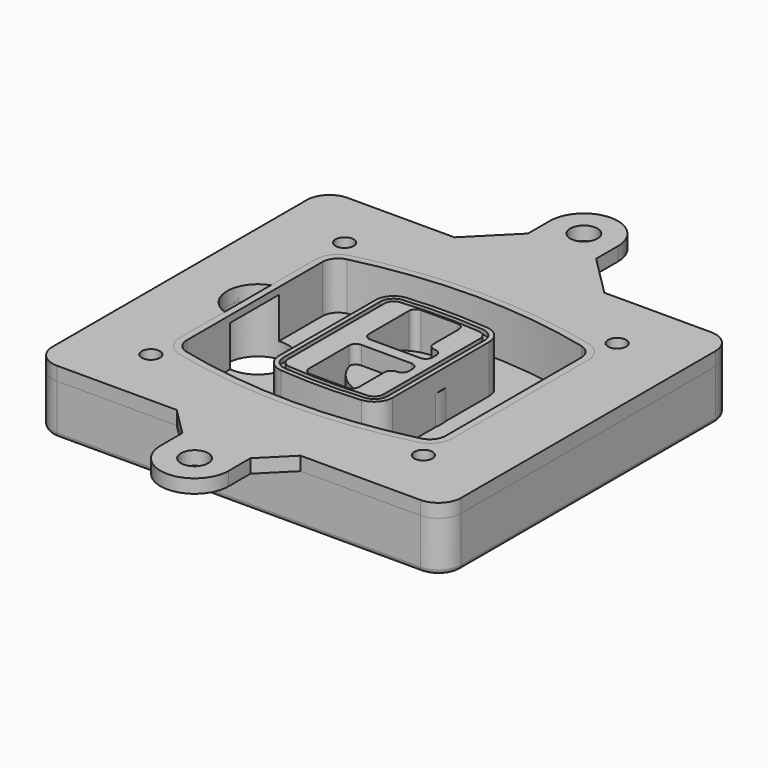
from build123d import *

# Parameters (mm, degrees)
F0_R      = 4
F1_DEPTH  = 25
F2_DEPTH  = 3
F3_DEPTH  = 18
F5_DEPTH  = 21
F6_DEPTH  = 2
F8_DEPTH  = 20
F9_DEPTH  = 16
F10_DEPTH = 25
F7_R      = 6
F7_R_2    = 4
F11_DEPTH = 6
F13_DEPTH = 9
F15_R     = 2
F16_R     = 4
F17_DEPTH = 3


# Not quite as in the source:
# - a feature of the source that left no trace in its solid (it failed there, or was rolled back) is left out
# - a feature names something its author has since deleted; it is built from what else it names


with BuildPart() as f1:
    # F0 (on Top) → F1 (new body)
    with BuildSketch(Plane.XY):
        with BuildLine():
            ThreePointArc((-90, -70), (-87.0710678119, -77.0710678119), (-80, -80))
            Line((-80, -80), (80, -80))
            ThreePointArc((80, -80), (87.0710678119, -77.0710678119), (90, -70))
            Line((90, -70), (90, 70))
            ThreePointArc((90, 70), (87.0710678119, 77.0710678119), (80, 80))
            Line((80, 80), (-80, 80))
            ThreePointArc((-80, 80), (-87.0710678119, 77.0710678119), (-90, 70))
            Line((-90, 70), (-90, -70))
        make_face()
        with Locations((-60, -53.3333333333)):
            Circle(F0_R, mode=Mode.SUBTRACT)
        with Locations((60, -53.3333333333)):
            Circle(F0_R, mode=Mode.SUBTRACT)
        with Locations((-60, 53.3333333333)):
            Circle(F0_R, mode=Mode.SUBTRACT)
        with BuildLine():
            ThreePointArc((-64, 37.2990447398), (-61.0143011354, 45.9411029726), (-53.3306899286, 50.8970778549))
            ThreePointArc((-53.3306899286, 50.8970778549), (0, 57.3333333333), (53.3306899286, 50.8970778549))
            ThreePointArc((53.3306899286, 50.8970778549), (61.0143011354, 45.9411029726), (64, 37.2990447398))
            Line((64, 37.2990447398), (64, -37.2990447398))
            ThreePointArc((64, -37.2990447398), (61.0143011354, -45.9411029726), (53.3306899286, -50.8970778549))
            ThreePointArc((53.3306899286, -50.8970778549), (0, -57.3333333333), (-53.3306899286, -50.8970778549))
            ThreePointArc((-53.3306899286, -50.8970778549), (-61.0143011354, -45.9411029726), (-64, -37.2990447398))
            Line((-64, -37.2990447398), (-64, 37.2990447398))
        make_face(mode=Mode.SUBTRACT)
        with Locations((60, 53.3333333333)):
            Circle(F0_R, mode=Mode.SUBTRACT)
        with BuildLine():
            ThreePointArc((53.3306899286, 50.8970778549), (0, 57.3333333333), (-53.3306899286, 50.8970778549))
            ThreePointArc((-53.3306899286, 50.8970778549), (-61.0143011354, 45.9411029726), (-64, 37.2990447398))
            Line((-64, 37.2990447398), (-64, -37.2990447398))
            ThreePointArc((-64, -37.2990447398), (-61.0143011354, -45.9411029726), (-53.3306899286, -50.8970778549))
            ThreePointArc((-53.3306899286, -50.8970778549), (0, -57.3333333333), (53.3306899286, -50.8970778549))
            ThreePointArc((53.3306899286, -50.8970778549), (61.0143011354, -45.9411029726), (64, -37.2990447398))
            Line((64, -37.2990447398), (64, 37.2990447398))
            ThreePointArc((64, 37.2990447398), (61.0143011354, 45.9411029726), (53.3306899286, 50.8970778549))
        make_face()
        with BuildLine():
            Line((-60, -37.2990447398), (-60, 37.2990447398))
            ThreePointArc((-60, 37.2990447398), (-57.8673579538, 43.4719434775), (-52.3790642347, 47.0119255363))
            ThreePointArc((-52.3790642347, 47.0119255363), (0, 53.3333333333), (52.3790642347, 47.0119255363))
            ThreePointArc((52.3790642347, 47.0119255363), (57.8673579538, 43.4719434775), (60, 37.2990447398))
            Line((60, 37.2990447398), (60, -37.2990447398))
            ThreePointArc((60, -37.2990447398), (57.8673579538, -43.4719434775), (52.3790642347, -47.0119255363))
            ThreePointArc((52.3790642347, -47.0119255363), (0, -53.3333333333), (-52.3790642347, -47.0119255363))
            ThreePointArc((-52.3790642347, -47.0119255363), (-57.8673579538, -43.4719434775), (-60, -37.2990447398))
        make_face(mode=Mode.SUBTRACT)
        with BuildLine():
            ThreePointArc((-52.3790642347, 47.0119255363), (-57.8673579538, 43.4719434775), (-60, 37.2990447398))
            Line((-60, 37.2990447398), (-60, -37.2990447398))
            ThreePointArc((-60, -37.2990447398), (-57.8673579538, -43.4719434775), (-52.3790642347, -47.0119255363))
            ThreePointArc((-52.3790642347, -47.0119255363), (0, -53.3333333333), (52.3790642347, -47.0119255363))
            ThreePointArc((52.3790642347, -47.0119255363), (57.8673579538, -43.4719434775), (60, -37.2990447398))
            Line((60, -37.2990447398), (60, 37.2990447398))
            ThreePointArc((60, 37.2990447398), (57.8673579538, 43.4719434775), (52.3790642347, 47.0119255363))
            ThreePointArc((52.3790642347, 47.0119255363), (0, 53.3333333333), (-52.3790642347, 47.0119255363))
        make_face()
        with BuildLine():
            ThreePointArc((51.6653449643, 44.0980612973), (55.5071505677, 41.6200738562), (57, 37.2990447398))
            Line((57, 37.2990447398), (57, -37.2990447398))
            ThreePointArc((57, -37.2990447398), (55.5071505677, -41.6200738562), (51.6653449643, -44.0980612973))
            ThreePointArc((51.6653449643, -44.0980612973), (0, -50.3333333333), (-51.6653449643, -44.0980612973))
            ThreePointArc((-51.6653449643, -44.0980612973), (-55.5071505677, -41.6200738562), (-57, -37.2990447398))
            Line((-57, -37.2990447398), (-57, 37.2990447398))
            ThreePointArc((-57, 37.2990447398), (-55.5071505677, 41.6200738562), (-51.6653449643, 44.0980612973))
            ThreePointArc((-51.6653449643, 44.0980612973), (0, 50.3333333333), (51.6653449643, 44.0980612973))
        make_face(mode=Mode.SUBTRACT)
        with BuildLine():
            Line((57, -37.2990447398), (57, 37.2990447398))
            ThreePointArc((57, 37.2990447398), (55.5071505677, 41.6200738562), (51.6653449643, 44.0980612973))
            ThreePointArc((51.6653449643, 44.0980612973), (0, 50.3333333333), (-51.6653449643, 44.0980612973))
            ThreePointArc((-51.6653449643, 44.0980612973), (-55.5071505677, 41.6200738562), (-57, 37.2990447398))
            Line((-57, 37.2990447398), (-57, -37.2990447398))
            ThreePointArc((-57, -37.2990447398), (-55.5071505677, -41.6200738562), (-51.6653449643, -44.0980612973))
            ThreePointArc((-51.6653449643, -44.0980612973), (0, -50.3333333333), (51.6653449643, -44.0980612973))
            ThreePointArc((51.6653449643, -44.0980612973), (55.5071505677, -41.6200738562), (57, -37.2990447398))
        make_face()
    extrude(amount=-F1_DEPTH)

    # F0 (on Top) → F2 (join)
    with BuildSketch(Plane.XY):
        with BuildLine():
            ThreePointArc((-52.3790642347, 47.0119255363), (-57.8673579538, 43.4719434775), (-60, 37.2990447398))
            Line((-60, 37.2990447398), (-60, -37.2990447398))
            ThreePointArc((-60, -37.2990447398), (-57.8673579538, -43.4719434775), (-52.3790642347, -47.0119255363))
            ThreePointArc((-52.3790642347, -47.0119255363), (0, -53.3333333333), (52.3790642347, -47.0119255363))
            ThreePointArc((52.3790642347, -47.0119255363), (57.8673579538, -43.4719434775), (60, -37.2990447398))
            Line((60, -37.2990447398), (60, 37.2990447398))
            ThreePointArc((60, 37.2990447398), (57.8673579538, 43.4719434775), (52.3790642347, 47.0119255363))
            ThreePointArc((52.3790642347, 47.0119255363), (0, 53.3333333333), (-52.3790642347, 47.0119255363))
        make_face()
        with BuildLine():
            ThreePointArc((51.6653449643, 44.0980612973), (55.5071505677, 41.6200738562), (57, 37.2990447398))
            Line((57, 37.2990447398), (57, -37.2990447398))
            ThreePointArc((57, -37.2990447398), (55.5071505677, -41.6200738562), (51.6653449643, -44.0980612973))
            ThreePointArc((51.6653449643, -44.0980612973), (0, -50.3333333333), (-51.6653449643, -44.0980612973))
            ThreePointArc((-51.6653449643, -44.0980612973), (-55.5071505677, -41.6200738562), (-57, -37.2990447398))
            Line((-57, -37.2990447398), (-57, 37.2990447398))
            ThreePointArc((-57, 37.2990447398), (-55.5071505677, 41.6200738562), (-51.6653449643, 44.0980612973))
            ThreePointArc((-51.6653449643, 44.0980612973), (0, 50.3333333333), (51.6653449643, 44.0980612973))
        make_face(mode=Mode.SUBTRACT)
    extrude(amount=F2_DEPTH)

    # F0 (on Top) → F3 (cut)
    with BuildSketch(Plane.XY):
        with BuildLine():
            Line((57, -37.2990447398), (57, 37.2990447398))
            ThreePointArc((57, 37.2990447398), (55.5071505677, 41.6200738562), (51.6653449643, 44.0980612973))
            ThreePointArc((51.6653449643, 44.0980612973), (0, 50.3333333333), (-51.6653449643, 44.0980612973))
            ThreePointArc((-51.6653449643, 44.0980612973), (-55.5071505677, 41.6200738562), (-57, 37.2990447398))
            Line((-57, 37.2990447398), (-57, -37.2990447398))
            ThreePointArc((-57, -37.2990447398), (-55.5071505677, -41.6200738562), (-51.6653449643, -44.0980612973))
            ThreePointArc((-51.6653449643, -44.0980612973), (0, -50.3333333333), (51.6653449643, -44.0980612973))
            ThreePointArc((51.6653449643, -44.0980612973), (55.5071505677, -41.6200738562), (57, -37.2990447398))
        make_face()
    extrude(amount=-F3_DEPTH, mode=Mode.SUBTRACT)

    # F4 (on face) → F5 (join, through all)
    with BuildSketch(Plane.XY.offset(3)):
        with BuildLine():
            ThreePointArc((-25, -26.587695628), (-22.8992979869, -31.9912392117), (-17.7004291845, -34.5569740744))
            ThreePointArc((-17.7004291845, -34.5569740744), (0, -35.3333333333), (17.7004291845, -34.5569740744))
            ThreePointArc((17.7004291845, -34.5569740744), (22.8992979869, -31.9912392117), (25, -26.587695628))
            Line((25, -26.587695628), (25, 26.587695628))
            ThreePointArc((25, 26.587695628), (22.8992979869, 31.9912392117), (17.7004291845, 34.5569740744))
            ThreePointArc((17.7004291845, 34.5569740744), (0, 35.3333333333), (-17.7004291845, 34.5569740744))
            ThreePointArc((-17.7004291845, 34.5569740744), (-22.8992979869, 31.9912392117), (-25, 26.587695628))
            Line((-25, 26.587695628), (-25, -26.587695628))
        make_face()
        with BuildLine():
            ThreePointArc((17.5253218884, 32.5646544628), (21.4244734902, 30.6403533158), (23, 26.587695628))
            Line((23, 26.587695628), (23, -26.587695628))
            ThreePointArc((23, -26.587695628), (21.4244734902, -30.6403533158), (17.5253218884, -32.5646544628))
            ThreePointArc((17.5253218884, -32.5646544628), (0, -33.3333333333), (-17.5253218884, -32.5646544628))
            ThreePointArc((-17.5253218884, -32.5646544628), (-21.4244734902, -30.6403533158), (-23, -26.587695628))
            Line((-23, -26.587695628), (-23, 26.587695628))
            ThreePointArc((-23, 26.587695628), (-21.4244734902, 30.6403533158), (-17.5253218884, 32.5646544628))
            ThreePointArc((-17.5253218884, 32.5646544628), (0, 33.3333333333), (17.5253218884, 32.5646544628))
        make_face(mode=Mode.SUBTRACT)
        with BuildLine():
            Line((23, -26.587695628), (23, 26.587695628))
            ThreePointArc((23, 26.587695628), (21.4244734902, 30.6403533158), (17.5253218884, 32.5646544628))
            ThreePointArc((17.5253218884, 32.5646544628), (0, 33.3333333333), (-17.5253218884, 32.5646544628))
            ThreePointArc((-17.5253218884, 32.5646544628), (-21.4244734902, 30.6403533158), (-23, 26.587695628))
            Line((-23, 26.587695628), (-23, -26.587695628))
            ThreePointArc((-23, -26.587695628), (-21.4244734902, -30.6403533158), (-17.5253218884, -32.5646544628))
            ThreePointArc((-17.5253218884, -32.5646544628), (0, -33.3333333333), (17.5253218884, -32.5646544628))
            ThreePointArc((17.5253218884, -32.5646544628), (21.4244734902, -30.6403533158), (23, -26.587695628))
        make_face()
        with BuildLine():
            ThreePointArc((17.3502145923, 30.5723348512), (19.9496489934, 29.2894674198), (21, 26.587695628))
            Line((21, 26.587695628), (21, -26.587695628))
            ThreePointArc((21, -26.587695628), (19.9496489934, -29.2894674198), (17.3502145923, -30.5723348512))
            ThreePointArc((17.3502145923, -30.5723348512), (0, -31.3333333333), (-17.3502145923, -30.5723348512))
            ThreePointArc((-17.3502145923, -30.5723348512), (-19.9496489934, -29.2894674198), (-21, -26.587695628))
            Line((-21, -26.587695628), (-21, 26.587695628))
            ThreePointArc((-21, 26.587695628), (-19.9496489934, 29.2894674198), (-17.3502145923, 30.5723348512))
            ThreePointArc((-17.3502145923, 30.5723348512), (0, 31.3333333333), (17.3502145923, 30.5723348512))
        make_face(mode=Mode.SUBTRACT)
        with BuildLine():
            Line((21, -26.587695628), (21, 26.587695628))
            ThreePointArc((21, 26.587695628), (19.9496489934, 29.2894674198), (17.3502145923, 30.5723348512))
            ThreePointArc((17.3502145923, 30.5723348512), (0, 31.3333333333), (-17.3502145923, 30.5723348512))
            ThreePointArc((-17.3502145923, 30.5723348512), (-19.9496489934, 29.2894674198), (-21, 26.587695628))
            Line((-21, 26.587695628), (-21, -26.587695628))
            ThreePointArc((-21, -26.587695628), (-19.9496489934, -29.2894674198), (-17.3502145923, -30.5723348512))
            ThreePointArc((-17.3502145923, -30.5723348512), (0, -31.3333333333), (17.3502145923, -30.5723348512))
            ThreePointArc((17.3502145923, -30.5723348512), (19.9496489934, -29.2894674198), (21, -26.587695628))
        make_face()
        with BuildLine():
            Line((-8, -2.5), (14, -2.5))
            ThreePointArc((14, -2.5), (16.1213203436, -3.3786796564), (17, -5.5))
            Line((17, -5.5), (17, -7.5))
            ThreePointArc((17, -7.5), (16.1213203436, -9.6213203436), (14, -10.5))
            ThreePointArc((14, -10.5), (11.8786796564, -11.3786796564), (11, -13.5))
            Line((11, -13.5), (11, -27.5))
            ThreePointArc((11, -27.5), (10.1213203436, -29.6213203436), (8, -30.5))
            Line((8, -30.5), (-8, -30.5))
            ThreePointArc((-8, -30.5), (-10.1213203436, -29.6213203436), (-11, -27.5))
            Line((-11, -27.5), (-11, -5.5))
            ThreePointArc((-11, -5.5), (-10.1213203436, -3.3786796564), (-8, -2.5))
        make_face(mode=Mode.SUBTRACT)
        with BuildLine():
            ThreePointArc((-8, 2.5), (-10.1213203436, 3.3786796564), (-11, 5.5))
            Line((-11, 5.5), (-11, 27.5))
            ThreePointArc((-11, 27.5), (-10.1213203436, 29.6213203436), (-8, 30.5))
            Line((-8, 30.5), (8, 30.5))
            ThreePointArc((8, 30.5), (10.1213203436, 29.6213203436), (11, 27.5))
            Line((11, 27.5), (11, 13.5))
            ThreePointArc((11, 13.5), (11.8786796564, 11.3786796564), (14, 10.5))
            ThreePointArc((14, 10.5), (16.1213203436, 9.6213203436), (17, 7.5))
            Line((17, 7.5), (17, 5.5))
            ThreePointArc((17, 5.5), (16.1213203436, 3.3786796564), (14, 2.5))
            Line((14, 2.5), (-8, 2.5))
        make_face(mode=Mode.SUBTRACT)
    extrude(amount=-F5_DEPTH)

    # F4 (on face) → F6 (cut)
    with BuildSketch(Plane.XY.offset(3)):
        with BuildLine():
            Line((23, -26.587695628), (23, 26.587695628))
            ThreePointArc((23, 26.587695628), (21.4244734902, 30.6403533158), (17.5253218884, 32.5646544628))
            ThreePointArc((17.5253218884, 32.5646544628), (0, 33.3333333333), (-17.5253218884, 32.5646544628))
            ThreePointArc((-17.5253218884, 32.5646544628), (-21.4244734902, 30.6403533158), (-23, 26.587695628))
            Line((-23, 26.587695628), (-23, -26.587695628))
            ThreePointArc((-23, -26.587695628), (-21.4244734902, -30.6403533158), (-17.5253218884, -32.5646544628))
            ThreePointArc((-17.5253218884, -32.5646544628), (0, -33.3333333333), (17.5253218884, -32.5646544628))
            ThreePointArc((17.5253218884, -32.5646544628), (21.4244734902, -30.6403533158), (23, -26.587695628))
        make_face()
        with BuildLine():
            ThreePointArc((17.3502145923, 30.5723348512), (19.9496489934, 29.2894674198), (21, 26.587695628))
            Line((21, 26.587695628), (21, -26.587695628))
            ThreePointArc((21, -26.587695628), (19.9496489934, -29.2894674198), (17.3502145923, -30.5723348512))
            ThreePointArc((17.3502145923, -30.5723348512), (0, -31.3333333333), (-17.3502145923, -30.5723348512))
            ThreePointArc((-17.3502145923, -30.5723348512), (-19.9496489934, -29.2894674198), (-21, -26.587695628))
            Line((-21, -26.587695628), (-21, 26.587695628))
            ThreePointArc((-21, 26.587695628), (-19.9496489934, 29.2894674198), (-17.3502145923, 30.5723348512))
            ThreePointArc((-17.3502145923, 30.5723348512), (0, 31.3333333333), (17.3502145923, 30.5723348512))
        make_face(mode=Mode.SUBTRACT)
    extrude(amount=-F6_DEPTH, mode=Mode.SUBTRACT)

    # F7 (on face) → F8 (join)
    with BuildSketch(Plane(origin=(0, 0, -25), x_dir=(1, 0, 0), z_dir=(0, 0, -1))):
        with BuildLine():
            ThreePointArc((-6.71157564, 0), (6.7567035675, 13.4682792075), (20.224982775, 0))
            Line((20.224982775, 0), (25.224982775, 0))
            ThreePointArc((25.224982775, 0), (6.7567035675, 18.4682792075), (-11.71157564, 0))
            Line((-11.71157564, 0), (-6.71157564, 0))
        make_face()
        with BuildLine():
            Line((-6.71157564, 0), (20.224982775, 0))
            ThreePointArc((20.224982775, 0), (6.7567035675, 13.4682792075), (-6.71157564, 0))
        make_face()
        with BuildLine():
            ThreePointArc((-6.71157564, 0), (6.7567035675, -13.4682792075), (20.224982775, 0))
            Line((20.224982775, 0), (-6.71157564, 0))
        make_face()
        with BuildLine():
            Line((25.224982775, 0), (20.224982775, 0))
            ThreePointArc((20.224982775, 0), (6.7567035675, -13.4682792075), (-6.71157564, 0))
            Line((-6.71157564, 0), (-11.71157564, 0))
            ThreePointArc((-11.71157564, 0), (6.7567035675, -18.4682792075), (25.224982775, 0))
        make_face()
    extrude(amount=-F8_DEPTH)

    # F7 (on face) → F9 (cut)
    with BuildSketch(Plane(origin=(0, 0, -25), x_dir=(1, 0, 0), z_dir=(0, 0, -1))):
        with BuildLine():
            Line((-6.71157564, 0), (20.224982775, 0))
            ThreePointArc((20.224982775, 0), (6.7567035675, 13.4682792075), (-6.71157564, 0))
        make_face()
        with BuildLine():
            ThreePointArc((-6.71157564, 0), (6.7567035675, -13.4682792075), (20.224982775, 0))
            Line((20.224982775, 0), (-6.71157564, 0))
        make_face()
    extrude(amount=-F9_DEPTH, mode=Mode.SUBTRACT)

    # F7 (on face) → F10 (cut)
    with BuildSketch(Plane(origin=(0, 0, -25), x_dir=(1, 0, 0), z_dir=(0, 0, -1))):
        with BuildLine():
            Line((-69.0318229325, 0), (-42.0952645175, 0))
            ThreePointArc((-42.0952645175, 0), (-55.563543725, 13.4682792075), (-69.0318229325, 0))
        make_face()
        with BuildLine():
            ThreePointArc((-69.0318229325, 0), (-55.563543725, -13.4682792075), (-42.0952645175, 0))
            Line((-42.0952645175, 0), (-69.0318229325, 0))
        make_face()
    extrude(amount=-F10_DEPTH, mode=Mode.SUBTRACT)

    # F7 (on face) → F11 (cut)
    with BuildSketch(Plane(origin=(0, 0, -25), x_dir=(1, 0, 0), z_dir=(0, 0, -1))):
        with Locations((60, -53.3333333333)):
            Circle(F7_R)
        with Locations((60, -53.3333333333)):
            Circle(F7_R_2, mode=Mode.SUBTRACT)
        with Locations((60, -53.3333333333)):
            Circle(F7_R)
        with Locations((60, -53.3333333333)):
            Circle(F7_R_2, mode=Mode.SUBTRACT)
        with Locations((-60, -53.3333333333)):
            Circle(F7_R)
        with Locations((-60, -53.3333333333)):
            Circle(F7_R_2, mode=Mode.SUBTRACT)
        with Locations((-60, -53.3333333333)):
            Circle(F7_R)
        with Locations((-60, -53.3333333333)):
            Circle(F7_R_2, mode=Mode.SUBTRACT)
        with Locations((-60, 53.3333333333)):
            Circle(F7_R)
        with Locations((-60, 53.3333333333)):
            Circle(F7_R_2, mode=Mode.SUBTRACT)
        with Locations((-60, 53.3333333333)):
            Circle(F7_R)
        with Locations((-60, 53.3333333333)):
            Circle(F7_R_2, mode=Mode.SUBTRACT)
        with Locations((60, 53.3333333333)):
            Circle(F7_R)
        with Locations((60, 53.3333333333)):
            Circle(F7_R_2, mode=Mode.SUBTRACT)
        with Locations((60, 53.3333333333)):
            Circle(F7_R)
        with Locations((60, 53.3333333333)):
            Circle(F7_R_2, mode=Mode.SUBTRACT)
    extrude(amount=-F11_DEPTH, mode=Mode.SUBTRACT)

    # F12 (on face) → F13 (cut, through all)
    with BuildSketch(Plane(origin=(0, 0, -9), x_dir=(1, 0, 0), z_dir=(0, 0, -1))):
        with BuildLine():
            ThreePointArc((20.224982775, 0), (20.1663399806, 1.2554664788), (19.9909222755, 2.5))
            Line((19.9909222755, 2.5), (14, 2.5))
            ThreePointArc((14, 2.5), (16.1213203436, 3.3786796564), (17, 5.5))
            Line((17, 5.5), (17, 7.5))
            ThreePointArc((17, 7.5), (16.1213203436, 9.6213203436), (14, 10.5))
            ThreePointArc((14, 10.5), (12.1627255951, 11.1284134507), (11.0951631559, 12.750384826))
            ThreePointArc((11.0951631559, 12.750384826), (11.0476113807, 12.7664660322), (11, 12.7823698976))
            Line((11, 12.7823698976), (11, -12.7823698976))
            ThreePointArc((11, -12.7823698976), (11.0476113807, -12.7664660322), (11.0951631559, -12.750384826))
            ThreePointArc((11.0951631559, -12.750384826), (12.1627255951, -11.1284134507), (14, -10.5))
            ThreePointArc((14, -10.5), (16.1213203436, -9.6213203436), (17, -7.5))
            Line((17, -7.5), (17, -5.5))
            ThreePointArc((17, -5.5), (16.1213203436, -3.3786796564), (14, -2.5))
            Line((14, -2.5), (19.9909222755, -2.5))
            ThreePointArc((19.9909222755, -2.5), (20.1663399806, -1.2554664788), (20.224982775, 0))
        make_face()
    extrude(amount=F13_DEPTH, mode=Mode.SUBTRACT)

    # F15
    f15_edges = [f1.edges().sort_by_distance(p)[0] for p in [
        (0, -80, -25),
        (-87.071068, -77.071068, -25),
        (-90, 0, -25),
        (-87.071068, 77.071068, -25),
        (87.071068, -77.071068, -25),
        (0, 80, -25),
        (90, 0, -25),
        (87.071068, 77.071068, -25),
    ]]
    fillet(f15_edges, radius=F15_R)


with BuildPart() as f17:
    # F16 (on face) → F17 (new body, symmetric)
    with BuildSketch(Plane.XY):
        with BuildLine():
            Line((-15, 98), (-33, 80))
            Line((-33, 80), (0, 80))
            Line((0, 80), (33, 80))
            Line((33, 80), (15, 98))
            Line((15, 98), (15, 110))
            ThreePointArc((15, 110), (0, 125), (-15, 110))
            Line((-15, 110), (-15, 98))
        make_face()
        with BuildLine():
            ThreePointArc((6, 110), (4.2426406871, 105.7573593129), (0, 104))
            ThreePointArc((0, 104), (-4.2426406871, 114.2426406871), (6, 110))
        make_face(mode=Mode.SUBTRACT)
        with BuildLine():
            Line((-33, 80), (-80, 80))
            ThreePointArc((-80, 80), (-87.0710678119, 77.0710678119), (-90, 70))
            Line((-90, 70), (-90, -70))
            ThreePointArc((-90, -70), (-87.0710678119, -77.0710678119), (-80, -80))
            Line((-80, -80), (-27.25, -80))
            Line((-27.25, -80), (0, -80))
            Line((0, -80), (27.25, -80))
            Line((27.25, -80), (80, -80))
            ThreePointArc((80, -80), (87.0710678119, -77.0710678119), (90, -70))
            Line((90, -70), (90, 70))
            ThreePointArc((90, 70), (87.0710678119, 77.0710678119), (80, 80))
            Line((80, 80), (33, 80))
            Line((33, 80), (0, 80))
            Line((0, 80), (-33, 80))
        make_face()
        with Locations((-60, -53.3333333333)):
            Circle(F16_R, mode=Mode.SUBTRACT)
        with BuildLine():
            ThreePointArc((-52.3790642347, 47.0119255363), (0, 53.3333333333), (52.3790642347, 47.0119255363))
            ThreePointArc((52.3790642347, 47.0119255363), (57.8673579538, 43.4719434775), (60, 37.2990447398))
            Line((60, 37.2990447398), (60, -37.2990447398))
            ThreePointArc((60, -37.2990447398), (57.8673579538, -43.4719434775), (52.3790642347, -47.0119255363))
            ThreePointArc((52.3790642347, -47.0119255363), (0, -53.3333333333), (-52.3790642347, -47.0119255363))
            ThreePointArc((-52.3790642347, -47.0119255363), (-57.8673579538, -43.4719434775), (-60, -37.2990447398))
            Line((-60, -37.2990447398), (-60, -12.7166190685))
            ThreePointArc((-60, -12.7166190685), (-66.5441169481, -7.798817635), (-69.0318229325, 0))
            ThreePointArc((-69.0318229325, 0), (-66.5441169481, 7.798817635), (-60, 12.7166190685))
            Line((-60, 12.7166190685), (-60, 37.2990447398))
            ThreePointArc((-60, 37.2990447398), (-57.8673579538, 43.4719434775), (-52.3790642347, 47.0119255363))
        make_face(mode=Mode.SUBTRACT)
        with Locations((60, -53.3333333333)):
            Circle(F16_R, mode=Mode.SUBTRACT)
        with Locations((-60, 53.3333333333)):
            Circle(F16_R, mode=Mode.SUBTRACT)
        with Locations((60, 53.3333333333)):
            Circle(F16_R, mode=Mode.SUBTRACT)
        with BuildLine():
            Line((0, -80), (-27.25, -80))
            Line((-27.25, -80), (-15, -92.25))
            Line((-15, -92.25), (-15, -104.25))
            ThreePointArc((-15, -104.25), (0, -119.25), (15, -104.25))
            Line((15, -104.25), (15, -92.25))
            Line((15, -92.25), (27.25, -80))
            Line((27.25, -80), (0, -80))
        make_face()
        with BuildLine():
            ThreePointArc((6, -104.25), (-4.2426406871, -108.4926406871), (0, -98.25))
            ThreePointArc((0, -98.25), (4.2426406871, -100.0073593129), (6, -104.25))
        make_face(mode=Mode.SUBTRACT)
        with BuildLine():
            Line((-33, 80), (-80, 80))
            ThreePointArc((-80, 80), (-87.0710678119, 77.0710678119), (-90, 70))
            Line((-90, 70), (-90, -70))
            ThreePointArc((-90, -70), (-87.0710678119, -77.0710678119), (-80, -80))
            Line((-80, -80), (-27.25, -80))
            Line((-27.25, -80), (0, -80))
            Line((0, -80), (27.25, -80))
            Line((27.25, -80), (80, -80))
            ThreePointArc((80, -80), (87.0710678119, -77.0710678119), (90, -70))
            Line((90, -70), (90, 70))
            ThreePointArc((90, 70), (87.0710678119, 77.0710678119), (80, 80))
            Line((80, 80), (33, 80))
            Line((33, 80), (0, 80))
            Line((0, 80), (-33, 80))
        make_face()
        with Locations((-60, -53.3333333333)):
            Circle(F16_R, mode=Mode.SUBTRACT)
        with BuildLine():
            ThreePointArc((-52.3790642347, 47.0119255363), (0, 53.3333333333), (52.3790642347, 47.0119255363))
            ThreePointArc((52.3790642347, 47.0119255363), (57.8673579538, 43.4719434775), (60, 37.2990447398))
            Line((60, 37.2990447398), (60, -37.2990447398))
            ThreePointArc((60, -37.2990447398), (57.8673579538, -43.4719434775), (52.3790642347, -47.0119255363))
            ThreePointArc((52.3790642347, -47.0119255363), (0, -53.3333333333), (-52.3790642347, -47.0119255363))
            ThreePointArc((-52.3790642347, -47.0119255363), (-57.8673579538, -43.4719434775), (-60, -37.2990447398))
            Line((-60, -37.2990447398), (-60, -12.7166190685))
            ThreePointArc((-60, -12.7166190685), (-66.5441169481, -7.798817635), (-69.0318229325, 0))
            ThreePointArc((-69.0318229325, 0), (-66.5441169481, 7.798817635), (-60, 12.7166190685))
            Line((-60, 12.7166190685), (-60, 37.2990447398))
            ThreePointArc((-60, 37.2990447398), (-57.8673579538, 43.4719434775), (-52.3790642347, 47.0119255363))
        make_face(mode=Mode.SUBTRACT)
        with Locations((60, -53.3333333333)):
            Circle(F16_R, mode=Mode.SUBTRACT)
        with Locations((-60, 53.3333333333)):
            Circle(F16_R, mode=Mode.SUBTRACT)
        with Locations((60, 53.3333333333)):
            Circle(F16_R, mode=Mode.SUBTRACT)
    extrude(amount=F17_DEPTH, both=True)


solid = Compound([f1.part, f17.part])
